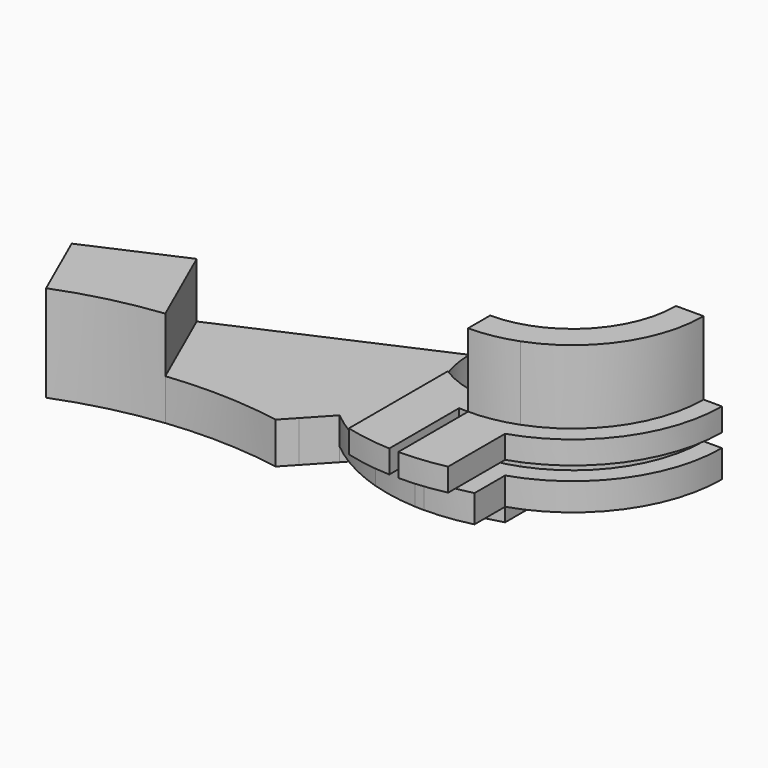
from build123d import *

# Parameters (mm, degrees)
F1_DEPTH = 3
F2_DEPTH = 4.5
F3_START = 4.5
F3_DEPTH = 2.5
F4_DEPTH = 15
F5_DEPTH = 9
F6_DEPTH = 1.5


with BuildPart() as f1:
    # F0 (on Top) → F1 (new body)
    with BuildSketch(Plane.XY):
        with BuildLine():
            Line((-28.99396, -19.230702), (-33.20482, -9.69463))
            Line((-33.20482, -9.69463), (-43.267447, -14.138003))
            Line((-43.267447, -14.138003), (-39.833932, -21.913668))
            ThreePointArc((-39.833932, -21.913668), (-34.501412, -20.218798), (-28.99396, -19.230702))
        make_face()
        with BuildLine():
            ThreePointArc((-15.304663, -18.161217), (-20.285575, -12.351435), (-23.160364, -5.259281))
            Line((-23.160364, -5.259281), (-33.20482, -9.69463))
            Line((-33.20482, -9.69463), (-28.99396, -19.230702))
            ThreePointArc((-28.99396, -19.230702), (-22.815941, -18.980633), (-16.665927, -19.619203))
            Line((-16.665927, -19.619203), (-15.304663, -18.161217))
        make_face()
        with BuildLine():
            ThreePointArc((-12.912473, -15.599056), (-17.426469, -10.3141), (-19.887562, -3.814104))
            Line((-19.887562, -3.814104), (-23.160364, -5.259281))
            ThreePointArc((-23.160364, -5.259281), (-20.285575, -12.351435), (-15.304663, -18.161217))
            Line((-15.304663, -18.161217), (-12.912473, -15.599056))
        make_face()
        with BuildLine():
            ThreePointArc((-10.176621, -12.668815), (-14.156447, -7.978565), (-16.107799, -2.145067))
            Line((-16.107799, -2.145067), (-19.887562, -3.814104))
            ThreePointArc((-19.887562, -3.814104), (-17.426469, -10.3141), (-12.912473, -15.599056))
            Line((-12.912473, -15.599056), (-10.176621, -12.668815))
        make_face()
        with BuildLine():
            ThreePointArc((-9.492159, -11.93572), (-13.33836, -7.392608), (-15.152334, -1.723161))
            Line((-15.152334, -1.723161), (-16.107799, -2.145067))
            ThreePointArc((-16.107799, -2.145067), (-14.156447, -7.978565), (-10.176621, -12.668815))
            Line((-10.176621, -12.668815), (-9.492159, -11.93572))
        make_face()
        with BuildLine():
            Line((-6, -15.101738), (-6, -14.020075))
            ThreePointArc((-6, -14.020075), (-7.815874, -13.094832), (-9.492159, -11.93572))
            Line((-9.492159, -11.93572), (-10.176621, -12.668815))
            ThreePointArc((-10.176621, -12.668815), (-8.179275, -14.041437), (-6, -15.101738))
        make_face()
        with BuildLine():
            ThreePointArc((-1, -15.217178), (-3.550812, -14.830854), (-6, -14.020075))
            Line((-6, -14.020075), (-6, -15.101738))
            ThreePointArc((-6, -15.101738), (-3.544317, -15.858762), (-1, -16.219202))
            Line((-1, -16.219202), (-1, -15.217178))
        make_face()
        with BuildLine():
            Line((5, -15.461646), (5, -14.40703))
            ThreePointArc((5, -14.40703), (2.535281, -15.037781), (0, -15.25))
            Line((0, -15.25), (0, -16.25))
            ThreePointArc((0, -16.25), (2.530884, -16.051702), (5, -15.461646))
        make_face()
        with BuildLine():
            Line((-6, -19.340695), (-6, -15.101738))
            ThreePointArc((-6, -15.101738), (-8.179275, -14.041437), (-10.176621, -12.668815))
            Line((-10.176621, -12.668815), (-12.912473, -15.599056))
            ThreePointArc((-12.912473, -15.599056), (-9.639521, -17.808485), (-6, -19.340695))
        make_face()
        with BuildLine():
            ThreePointArc((-1, -16.219202), (-3.544317, -15.858762), (-6, -15.101738))
            Line((-6, -15.101738), (-6, -19.340695))
            ThreePointArc((-6, -19.340695), (-3.527836, -19.940333), (-1, -20.225294))
            Line((-1, -20.225294), (-1, -16.219202))
        make_face()
        with BuildLine():
            Line((5, -19.623009), (5, -15.461646))
            ThreePointArc((5, -15.461646), (2.530884, -16.051702), (0, -16.25))
            Line((0, -16.25), (0, -20.25))
            ThreePointArc((0, -20.25), (2.519579, -20.092641), (5, -19.623009))
        make_face()
        with BuildLine():
            ThreePointArc((-6, -9.516433), (-9.850444, -5.434266), (-11.25, 0))
            Line((-11.25, 0), (-14.190712, -1.298536))
            ThreePointArc((-14.190712, -1.298536), (-11.649525, -8.20677), (-6, -12.925266))
            Line((-6, -12.925266), (-6, -9.516433))
        make_face()
        with BuildLine():
            ThreePointArc((-6, -12.925266), (-11.649525, -8.20677), (-14.190712, -1.298536))
            Line((-14.190712, -1.298536), (-15.152334, -1.723161))
            ThreePointArc((-15.152334, -1.723161), (-13.33836, -7.392608), (-9.492159, -11.93572))
            ThreePointArc((-9.492159, -11.93572), (-7.815874, -13.094832), (-6, -14.020075))
            Line((-6, -14.020075), (-6, -12.925266))
        make_face()
        with BuildLine():
            ThreePointArc((-1, -11.205467), (-3.600446, -10.658297), (-6, -9.516433))
            Line((-6, -9.516433), (-6, -12.925266))
            ThreePointArc((-6, -12.925266), (-3.5589, -13.798432), (-1, -14.214869))
            Line((-1, -14.214869), (-1, -11.205467))
        make_face()
        with BuildLine():
            ThreePointArc((-1, -14.214869), (-3.5589, -13.798432), (-6, -12.925266))
            Line((-6, -12.925266), (-6, -14.020075))
            ThreePointArc((-6, -14.020075), (-3.550812, -14.830854), (-1, -15.217178))
            Line((-1, -15.217178), (-1, -14.214869))
        make_face()
        with BuildLine():
            Line((5, -13.344006), (5, -10.077822))
            ThreePointArc((5, -10.077822), (2.567781, -10.953036), (0, -11.25))
            Line((0, -11.25), (0, -14.25))
            ThreePointArc((0, -14.25), (2.54071, -14.021672), (5, -13.344006))
        make_face()
        with BuildLine():
            Line((5, -14.40703), (5, -13.344006))
            ThreePointArc((5, -13.344006), (2.54071, -14.021672), (0, -14.25))
            Line((0, -14.25), (0, -15.25))
            ThreePointArc((0, -15.25), (2.535281, -15.037781), (5, -14.40703))
        make_face()
        with BuildLine():
            Line((14.25, 0), (11.25, 0))
            ThreePointArc((11.25, 0), (9.560662, -5.929271), (5, -10.077822))
            Line((5, -10.077822), (5, -13.344006))
            ThreePointArc((5, -13.344006), (11.711373, -8.118266), (14.25, 0))
        make_face()
        with BuildLine():
            Line((15.25, 0), (14.25, 0))
            ThreePointArc((14.25, 0), (11.711373, -8.118266), (5, -13.344006))
            Line((5, -13.344006), (5, -14.40703))
            ThreePointArc((5, -14.40703), (12.426031, -8.840602), (15.25, 0))
        make_face()
        with BuildLine():
            Line((16.25, 0), (15.25, 0))
            ThreePointArc((15.25, 0), (12.426031, -8.840602), (5, -14.40703))
            Line((5, -14.40703), (5, -15.461646))
            ThreePointArc((5, -15.461646), (13.139872, -9.560662), (16.25, 0))
        make_face()
        with BuildLine():
            Line((0, -20.25), (0, -16.25))
            ThreePointArc((0, -16.25), (-0.500237, -16.242299), (-1, -16.219202))
            Line((-1, -16.219202), (-1, -20.225294))
            ThreePointArc((-1, -20.225294), (-0.500153, -20.243822), (0, -20.25))
        make_face()
        with BuildLine():
            Line((0, -16.25), (0, -15.25))
            ThreePointArc((0, -15.25), (-0.500269, -15.241792), (-1, -15.217178))
            Line((-1, -15.217178), (-1, -16.219202))
            ThreePointArc((-1, -16.219202), (-0.500237, -16.242299), (0, -16.25))
        make_face()
        with BuildLine():
            Line((0, -15.25), (0, -14.25))
            ThreePointArc((0, -14.25), (-0.500308, -14.241215), (-1, -14.214869))
            Line((-1, -14.214869), (-1, -15.217178))
            ThreePointArc((-1, -15.217178), (-0.500269, -15.241792), (0, -15.25))
        make_face()
        with BuildLine():
            Line((0, -14.25), (0, -11.25))
            ThreePointArc((0, -11.25), (-0.500496, -11.238861), (-1, -11.205467))
            Line((-1, -11.205467), (-1, -14.214869))
            ThreePointArc((-1, -14.214869), (-0.500308, -14.241215), (0, -14.25))
        make_face()
    extrude(amount=F1_DEPTH)

    # F0 (on Top) → F2 (join)
    with BuildSketch(Plane.XY):
        with BuildLine():
            Line((14.25, 0), (11.25, 0))
            ThreePointArc((11.25, 0), (9.560662, -5.929271), (5, -10.077822))
            Line((5, -10.077822), (5, -13.344006))
            ThreePointArc((5, -13.344006), (11.711373, -8.118266), (14.25, 0))
        make_face()
        with BuildLine():
            Line((5, -13.344006), (5, -10.077822))
            ThreePointArc((5, -10.077822), (2.567781, -10.953036), (0, -11.25))
            Line((0, -11.25), (0, -14.25))
            ThreePointArc((0, -14.25), (2.54071, -14.021672), (5, -13.344006))
        make_face()
        with BuildLine():
            Line((0, -14.25), (0, -11.25))
            ThreePointArc((0, -11.25), (-0.500496, -11.238861), (-1, -11.205467))
            Line((-1, -11.205467), (-1, -14.214869))
            ThreePointArc((-1, -14.214869), (-0.500308, -14.241215), (0, -14.25))
        make_face()
        with BuildLine():
            ThreePointArc((-1, -11.205467), (-3.600446, -10.658297), (-6, -9.516433))
            Line((-6, -9.516433), (-6, -12.925266))
            ThreePointArc((-6, -12.925266), (-3.5589, -13.798432), (-1, -14.214869))
            Line((-1, -14.214869), (-1, -11.205467))
        make_face()
        with BuildLine():
            ThreePointArc((-1, -14.214869), (-3.5589, -13.798432), (-6, -12.925266))
            Line((-6, -12.925266), (-6, -14.020075))
            ThreePointArc((-6, -14.020075), (-3.550812, -14.830854), (-1, -15.217178))
            Line((-1, -15.217178), (-1, -14.214869))
        make_face()
        with BuildLine():
            ThreePointArc((-1, -15.217178), (-3.550812, -14.830854), (-6, -14.020075))
            Line((-6, -14.020075), (-6, -15.101738))
            ThreePointArc((-6, -15.101738), (-3.544317, -15.858762), (-1, -16.219202))
            Line((-1, -16.219202), (-1, -15.217178))
        make_face()
        with BuildLine():
            ThreePointArc((-1, -16.219202), (-3.544317, -15.858762), (-6, -15.101738))
            Line((-6, -15.101738), (-6, -19.340695))
            ThreePointArc((-6, -19.340695), (-3.527836, -19.940333), (-1, -20.225294))
            Line((-1, -20.225294), (-1, -16.219202))
        make_face()
    extrude(amount=F2_DEPTH)

    # F0 (on Top) → F3 (join)
    with BuildSketch(Plane.XY.offset(F3_START)):
        with BuildLine():
            Line((14.25, 0), (11.25, 0))
            ThreePointArc((11.25, 0), (9.560662, -5.929271), (5, -10.077822))
            Line((5, -10.077822), (5, -13.344006))
            ThreePointArc((5, -13.344006), (11.711373, -8.118266), (14.25, 0))
        make_face()
        with BuildLine():
            Line((15.25, 0), (14.25, 0))
            ThreePointArc((14.25, 0), (11.711373, -8.118266), (5, -13.344006))
            Line((5, -13.344006), (5, -14.40703))
            ThreePointArc((5, -14.40703), (12.426031, -8.840602), (15.25, 0))
        make_face()
        with BuildLine():
            Line((16.25, 0), (15.25, 0))
            ThreePointArc((15.25, 0), (12.426031, -8.840602), (5, -14.40703))
            Line((5, -14.40703), (5, -15.461646))
            ThreePointArc((5, -15.461646), (13.139872, -9.560662), (16.25, 0))
        make_face()
        with BuildLine():
            Line((5, -13.344006), (5, -10.077822))
            ThreePointArc((5, -10.077822), (2.567781, -10.953036), (0, -11.25))
            Line((0, -11.25), (0, -14.25))
            ThreePointArc((0, -14.25), (2.54071, -14.021672), (5, -13.344006))
        make_face()
        with BuildLine():
            Line((5, -14.40703), (5, -13.344006))
            ThreePointArc((5, -13.344006), (2.54071, -14.021672), (0, -14.25))
            Line((0, -14.25), (0, -15.25))
            ThreePointArc((0, -15.25), (2.535281, -15.037781), (5, -14.40703))
        make_face()
        with BuildLine():
            Line((5, -15.461646), (5, -14.40703))
            ThreePointArc((5, -14.40703), (2.535281, -15.037781), (0, -15.25))
            Line((0, -15.25), (0, -16.25))
            ThreePointArc((0, -16.25), (2.530884, -16.051702), (5, -15.461646))
        make_face()
        with BuildLine():
            Line((5, -19.623009), (5, -15.461646))
            ThreePointArc((5, -15.461646), (2.530884, -16.051702), (0, -16.25))
            Line((0, -16.25), (0, -20.25))
            ThreePointArc((0, -20.25), (2.519579, -20.092641), (5, -19.623009))
        make_face()
        with BuildLine():
            Line((0, -14.25), (0, -11.25))
            ThreePointArc((0, -11.25), (-0.500496, -11.238861), (-1, -11.205467))
            Line((-1, -11.205467), (-1, -14.214869))
            ThreePointArc((-1, -14.214869), (-0.500308, -14.241215), (0, -14.25))
        make_face()
        with BuildLine():
            ThreePointArc((-1, -11.205467), (-3.600446, -10.658297), (-6, -9.516433))
            Line((-6, -9.516433), (-6, -12.925266))
            ThreePointArc((-6, -12.925266), (-3.5589, -13.798432), (-1, -14.214869))
            Line((-1, -14.214869), (-1, -11.205467))
        make_face()
        with BuildLine():
            ThreePointArc((-1, -14.214869), (-3.5589, -13.798432), (-6, -12.925266))
            Line((-6, -12.925266), (-6, -14.020075))
            ThreePointArc((-6, -14.020075), (-3.550812, -14.830854), (-1, -15.217178))
            Line((-1, -15.217178), (-1, -14.214869))
        make_face()
        with BuildLine():
            ThreePointArc((-1, -15.217178), (-3.550812, -14.830854), (-6, -14.020075))
            Line((-6, -14.020075), (-6, -15.101738))
            ThreePointArc((-6, -15.101738), (-3.544317, -15.858762), (-1, -16.219202))
            Line((-1, -16.219202), (-1, -15.217178))
        make_face()
        with BuildLine():
            ThreePointArc((-1, -16.219202), (-3.544317, -15.858762), (-6, -15.101738))
            Line((-6, -15.101738), (-6, -19.340695))
            ThreePointArc((-6, -19.340695), (-3.527836, -19.940333), (-1, -20.225294))
            Line((-1, -20.225294), (-1, -16.219202))
        make_face()
        with BuildLine():
            Line((5, -23.21772), (5, -19.623009))
            ThreePointArc((5, -19.623009), (2.519579, -20.092641), (0, -20.25))
            Line((0, -20.25), (0, -23.75))
            ThreePointArc((0, -23.75), (2.514126, -23.616555), (5, -23.21772))
        make_face()
        with BuildLine():
            ThreePointArc((-1, -20.225294), (-3.527836, -19.940333), (-6, -19.340695))
            Line((-6, -19.340695), (-6, -22.979611))
            ThreePointArc((-6, -22.979611), (-3.519996, -23.487702), (-1, -23.728938))
            Line((-1, -23.728938), (-1, -20.225294))
        make_face()
    extrude(amount=F3_DEPTH)

    # F0 (on Top) → F4 (join)
    with BuildSketch(Plane.XY):
        with BuildLine():
            Line((14.25, 0), (11.25, 0))
            ThreePointArc((11.25, 0), (9.560662, -5.929271), (5, -10.077822))
            Line((5, -10.077822), (5, -13.344006))
            ThreePointArc((5, -13.344006), (11.711373, -8.118266), (14.25, 0))
        make_face()
        with BuildLine():
            Line((5, -13.344006), (5, -10.077822))
            ThreePointArc((5, -10.077822), (2.567781, -10.953036), (0, -11.25))
            Line((0, -11.25), (0, -14.25))
            ThreePointArc((0, -14.25), (2.54071, -14.021672), (5, -13.344006))
        make_face()
    extrude(amount=F4_DEPTH)

    # F0 (on Top) → F5 (join)
    with BuildSketch(Plane.XY):
        with BuildLine():
            Line((-28.99396, -19.230702), (-33.20482, -9.69463))
            Line((-33.20482, -9.69463), (-43.267447, -14.138003))
            Line((-43.267447, -14.138003), (-39.833932, -21.913668))
            ThreePointArc((-39.833932, -21.913668), (-34.501412, -20.218798), (-28.99396, -19.230702))
        make_face()
    extrude(amount=F5_DEPTH)

    # F0 (on Top) → F6 (join)
    with BuildSketch(Plane.XY):
        with BuildLine():
            Line((-28.99396, -19.230702), (-33.20482, -9.69463))
            Line((-33.20482, -9.69463), (-43.267447, -14.138003))
            Line((-43.267447, -14.138003), (-39.833932, -21.913668))
            ThreePointArc((-39.833932, -21.913668), (-34.501412, -20.218798), (-28.99396, -19.230702))
        make_face()
        with BuildLine():
            ThreePointArc((-15.304663, -18.161217), (-20.285575, -12.351435), (-23.160364, -5.259281))
            Line((-23.160364, -5.259281), (-33.20482, -9.69463))
            Line((-33.20482, -9.69463), (-28.99396, -19.230702))
            ThreePointArc((-28.99396, -19.230702), (-22.815941, -18.980633), (-16.665927, -19.619203))
            Line((-16.665927, -19.619203), (-15.304663, -18.161217))
        make_face()
        with BuildLine():
            ThreePointArc((-12.912473, -15.599056), (-17.426469, -10.3141), (-19.887562, -3.814104))
            Line((-19.887562, -3.814104), (-23.160364, -5.259281))
            ThreePointArc((-23.160364, -5.259281), (-20.285575, -12.351435), (-15.304663, -18.161217))
            Line((-15.304663, -18.161217), (-12.912473, -15.599056))
        make_face()
        with BuildLine():
            ThreePointArc((-10.176621, -12.668815), (-14.156447, -7.978565), (-16.107799, -2.145067))
            Line((-16.107799, -2.145067), (-19.887562, -3.814104))
            ThreePointArc((-19.887562, -3.814104), (-17.426469, -10.3141), (-12.912473, -15.599056))
            Line((-12.912473, -15.599056), (-10.176621, -12.668815))
        make_face()
        with BuildLine():
            ThreePointArc((-9.492159, -11.93572), (-13.33836, -7.392608), (-15.152334, -1.723161))
            Line((-15.152334, -1.723161), (-16.107799, -2.145067))
            ThreePointArc((-16.107799, -2.145067), (-14.156447, -7.978565), (-10.176621, -12.668815))
            Line((-10.176621, -12.668815), (-9.492159, -11.93572))
        make_face()
        with BuildLine():
            ThreePointArc((-6, -12.925266), (-11.649525, -8.20677), (-14.190712, -1.298536))
            Line((-14.190712, -1.298536), (-15.152334, -1.723161))
            ThreePointArc((-15.152334, -1.723161), (-13.33836, -7.392608), (-9.492159, -11.93572))
            ThreePointArc((-9.492159, -11.93572), (-7.815874, -13.094832), (-6, -14.020075))
            Line((-6, -14.020075), (-6, -12.925266))
        make_face()
        with BuildLine():
            ThreePointArc((-6, -9.516433), (-9.850444, -5.434266), (-11.25, 0))
            Line((-11.25, 0), (-14.190712, -1.298536))
            ThreePointArc((-14.190712, -1.298536), (-11.649525, -8.20677), (-6, -12.925266))
            Line((-6, -12.925266), (-6, -9.516433))
        make_face()
        with BuildLine():
            Line((-6, -15.101738), (-6, -14.020075))
            ThreePointArc((-6, -14.020075), (-7.815874, -13.094832), (-9.492159, -11.93572))
            Line((-9.492159, -11.93572), (-10.176621, -12.668815))
            ThreePointArc((-10.176621, -12.668815), (-8.179275, -14.041437), (-6, -15.101738))
        make_face()
        with BuildLine():
            ThreePointArc((-1, -11.205467), (-3.600446, -10.658297), (-6, -9.516433))
            Line((-6, -9.516433), (-6, -12.925266))
            ThreePointArc((-6, -12.925266), (-3.5589, -13.798432), (-1, -14.214869))
            Line((-1, -14.214869), (-1, -11.205467))
        make_face()
        with BuildLine():
            ThreePointArc((-1, -14.214869), (-3.5589, -13.798432), (-6, -12.925266))
            Line((-6, -12.925266), (-6, -14.020075))
            ThreePointArc((-6, -14.020075), (-3.550812, -14.830854), (-1, -15.217178))
            Line((-1, -15.217178), (-1, -14.214869))
        make_face()
        with BuildLine():
            ThreePointArc((-1, -15.217178), (-3.550812, -14.830854), (-6, -14.020075))
            Line((-6, -14.020075), (-6, -15.101738))
            ThreePointArc((-6, -15.101738), (-3.544317, -15.858762), (-1, -16.219202))
            Line((-1, -16.219202), (-1, -15.217178))
        make_face()
        with BuildLine():
            Line((5, -13.344006), (5, -10.077822))
            ThreePointArc((5, -10.077822), (2.567781, -10.953036), (0, -11.25))
            Line((0, -11.25), (0, -14.25))
            ThreePointArc((0, -14.25), (2.54071, -14.021672), (5, -13.344006))
        make_face()
        with BuildLine():
            Line((5, -14.40703), (5, -13.344006))
            ThreePointArc((5, -13.344006), (2.54071, -14.021672), (0, -14.25))
            Line((0, -14.25), (0, -15.25))
            ThreePointArc((0, -15.25), (2.535281, -15.037781), (5, -14.40703))
        make_face()
        with BuildLine():
            Line((5, -15.461646), (5, -14.40703))
            ThreePointArc((5, -14.40703), (2.535281, -15.037781), (0, -15.25))
            Line((0, -15.25), (0, -16.25))
            ThreePointArc((0, -16.25), (2.530884, -16.051702), (5, -15.461646))
        make_face()
        with BuildLine():
            Line((0, -16.25), (0, -15.25))
            ThreePointArc((0, -15.25), (-0.500269, -15.241792), (-1, -15.217178))
            Line((-1, -15.217178), (-1, -16.219202))
            ThreePointArc((-1, -16.219202), (-0.500237, -16.242299), (0, -16.25))
        make_face()
        with BuildLine():
            Line((0, -15.25), (0, -14.25))
            ThreePointArc((0, -14.25), (-0.500308, -14.241215), (-1, -14.214869))
            Line((-1, -14.214869), (-1, -15.217178))
            ThreePointArc((-1, -15.217178), (-0.500269, -15.241792), (0, -15.25))
        make_face()
        with BuildLine():
            Line((0, -14.25), (0, -11.25))
            ThreePointArc((0, -11.25), (-0.500496, -11.238861), (-1, -11.205467))
            Line((-1, -11.205467), (-1, -14.214869))
            ThreePointArc((-1, -14.214869), (-0.500308, -14.241215), (0, -14.25))
        make_face()
    extrude(amount=-F6_DEPTH)


solid = f1.part
